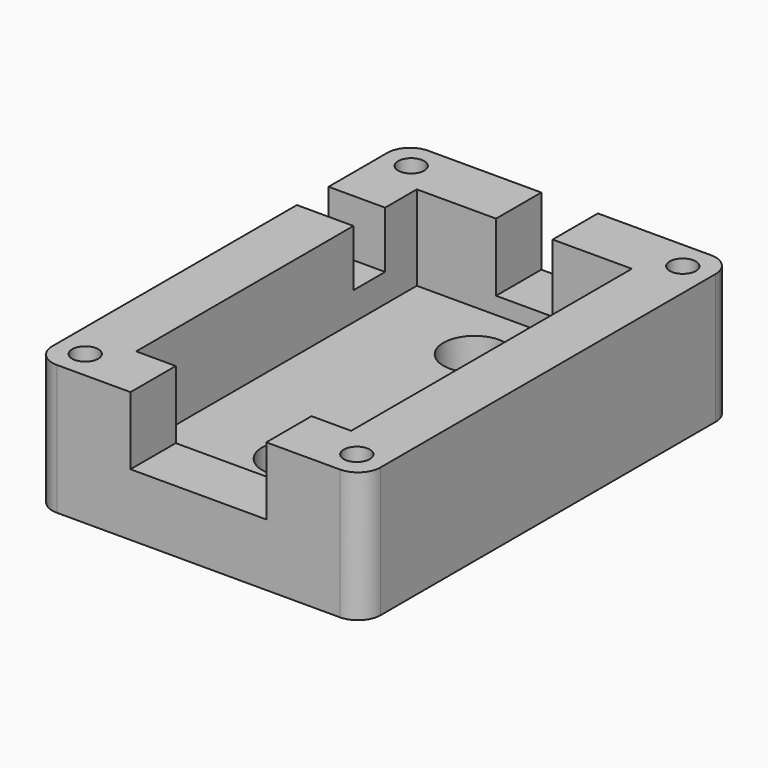
from build123d import *

# Parameters (mm, degrees)
F0_W           = 29
F0_H           = 41
F0_R           = 1.15
F0_W_2         = 19
F0_H_2         = 31
F1_DEPTH       = 7.5
F2_W           = 29
F2_H           = 41
F2_R           = 1.15
F2_W_2         = 19
F2_H_2         = 31
F3_DEPTH       = 4
F4_W           = 12
F4_H           = 5
F4_W_2         = 5
F5_DEPTH       = 6
F6_R           = 2
F8_D           = 2.9
F8_CBORE_D     = 5.5
F8_CBORE_DEPTH = 2.5
F9_W           = 5
F9_H           = 3.5
F10_DEPTH      = 5


with BuildPart() as f1:
    # F0 (on Top) → F1 (new body)
    with BuildSketch(Plane.XY):
        Rectangle(F0_W, F0_H)
        with Locations((-12, -18)):
            Circle(F0_R, mode=Mode.SUBTRACT)
        with Locations((12, -18)):
            Circle(F0_R, mode=Mode.SUBTRACT)
        with Locations((-12, 18)):
            Circle(F0_R, mode=Mode.SUBTRACT)
        Rectangle(F0_W_2, F0_H_2, mode=Mode.SUBTRACT)
        with Locations((12, 18)):
            Circle(F0_R, mode=Mode.SUBTRACT)
    extrude(amount=F1_DEPTH)

    # F2 (on face) → F3 (join)
    with BuildSketch(Plane(origin=(0, 0, 0), x_dir=(1, 0, 0), z_dir=(0, 0, -1))):
        Rectangle(F2_W, F2_H)
        with Locations((-12, -18)):
            Circle(F2_R, mode=Mode.SUBTRACT)
        with Locations((12, -18)):
            Circle(F2_R, mode=Mode.SUBTRACT)
        with Locations((-12, 18)):
            Circle(F2_R, mode=Mode.SUBTRACT)
        Rectangle(F2_W_2, F2_H_2, mode=Mode.SUBTRACT)
        with Locations((12, 18)):
            Circle(F2_R, mode=Mode.SUBTRACT)
        with Locations((-12, 18)):
            Circle(F2_R)
        with Locations((12, 18)):
            Circle(F2_R)
        with Locations((-12, -18)):
            Circle(F2_R)
        Rectangle(F2_W_2, F2_H_2)
        with Locations((12, -18)):
            Circle(F2_R)
    extrude(amount=F3_DEPTH)

    # F4 (on face) → F5 (cut)
    with BuildSketch(Plane.XY.offset(7.5)):
        with Locations((0, -18)):
            Rectangle(F4_W, F4_H)
        with Locations((0, 18)):
            Rectangle(F4_W_2, F4_H)
    extrude(amount=-F5_DEPTH, mode=Mode.SUBTRACT)

    # F6
    f6_edges = [f1.edges().sort_by_distance(p)[0] for p in [
        (-14.5, 20.5, 1.75),
        (14.5, 20.5, 1.75),
        (14.5, -20.5, 1.75),
        (-14.5, -20.5, 1.75),
    ]]
    fillet(f6_edges, radius=F6_R)

    # F8 (through all)
    with Locations(Plane.XY):
        with Locations((0, 10), (0, -10)):
            CounterBoreHole(F8_D / 2, F8_CBORE_D / 2, F8_CBORE_DEPTH)

    # F9 (on face) → F10 (cut)
    with BuildSketch(Plane.XY.offset(7.5)):
        with Locations((-12, 10.25)):
            Rectangle(F9_W, F9_H)
    extrude(amount=-F10_DEPTH, mode=Mode.SUBTRACT)


solid = f1.part
